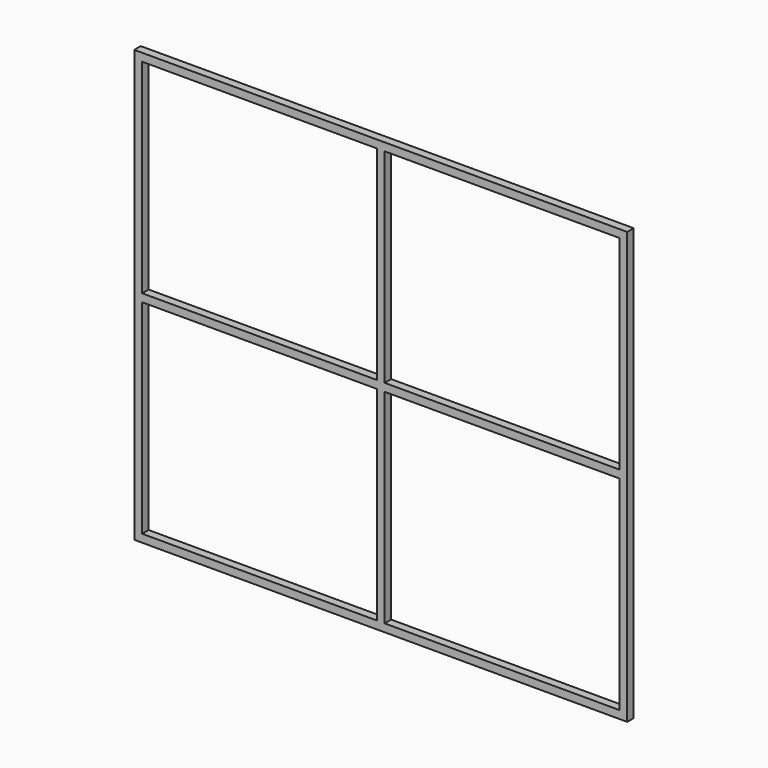
from build123d import *

# Parameters (mm, degrees)
F0_W     = 2000
F0_H     = 1750
F0_W_2   = 952
F0_H_2   = 32
F0_W_3   = 32
F0_H_3   = 827
F1_DEPTH = 33


with BuildPart() as f1:
    # F0 (on Front) → F1 (new body)
    with BuildSketch(Plane.XZ):
        with Locations((1000, 875)):
            Rectangle(F0_W, F0_H)
        Polygon((984, 32), (32, 32), (32, 859), (32, 891), (32, 1718), (984, 1718), (1016, 1718), (1968, 1718), (1968, 891), (1968, 859), (1968, 32), (1016, 32), align=None, mode=Mode.SUBTRACT)
        with Locations((508, 875)):
            Rectangle(F0_W_2, F0_H_2)
        with Locations((1000, 445.5)):
            Rectangle(F0_W_3, F0_H_3)
        with Locations((1000, 875)):
            Rectangle(F0_W_3, F0_H_2)
        with Locations((1000, 1304.5)):
            Rectangle(F0_W_3, F0_H_3)
        with Locations((1492, 875)):
            Rectangle(F0_W_2, F0_H_2)
    extrude(amount=F1_DEPTH)


solid = f1.part
